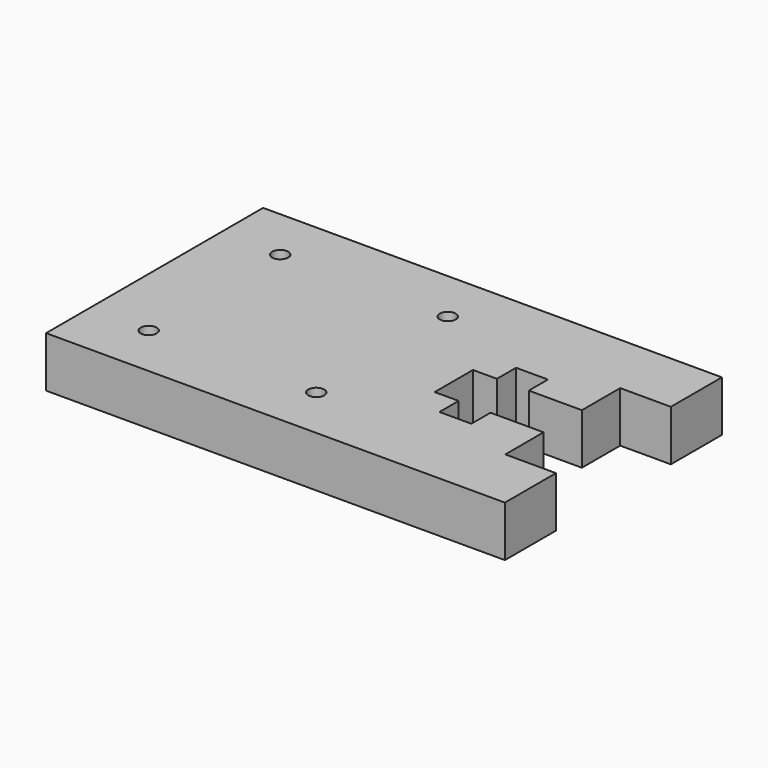
from build123d import *

# Parameters (mm, degrees)
F0_R     = 0.5
F1_DEPTH = 3.175


# Not quite as in the source:
# - a length typed as a fraction of an inch, garbled in the dataset ("3 / 203.2 mm" for 3/8 in), is restored


with BuildPart() as f1:
    # F0 (on Top) → F1 (new body)
    with BuildSketch(Plane.XY):
        Polygon((38.5022973402, 19.5465350598), (38.5022973402, 22.5465350598), (40.0022973402, 22.5465350598), (40.0022973402, 24.0465350598), (42.0022973402, 24.0465350598), (42.0022973402, 22.5465350598), (45.3272973402, 22.5465350598), (45.3272973402, 25.5465350598), (48.5022973402, 25.5465350598), (48.5022973402, 29.5465350598), (45.3272973402, 29.5465350598), (19.7522973402, 29.5465350598), (19.7522973402, 12.5465350598), (45.3272973402, 12.5465350598), (48.5022973402, 12.5465350598), (48.5022973402, 16.5465350598), (45.3272973402, 16.5465350598), (45.3272973402, 19.5465350598), (42.0022973402, 19.5465350598), (42.0022973402, 18.0465350598), (40.0022973402, 18.0465350598), (40.0022973402, 19.5465350598), align=None)
        with Locations((23.5022973402, 15.8965350598)):
            Circle(F0_R, mode=Mode.SUBTRACT)
        with Locations((34.0022973402, 15.8965350598)):
            Circle(F0_R, mode=Mode.SUBTRACT)
        with Locations((23.5022973402, 26.1965350598)):
            Circle(F0_R, mode=Mode.SUBTRACT)
        with Locations((34.0022973402, 26.1965350598)):
            Circle(F0_R, mode=Mode.SUBTRACT)
    extrude(amount=F1_DEPTH)


solid = f1.part
